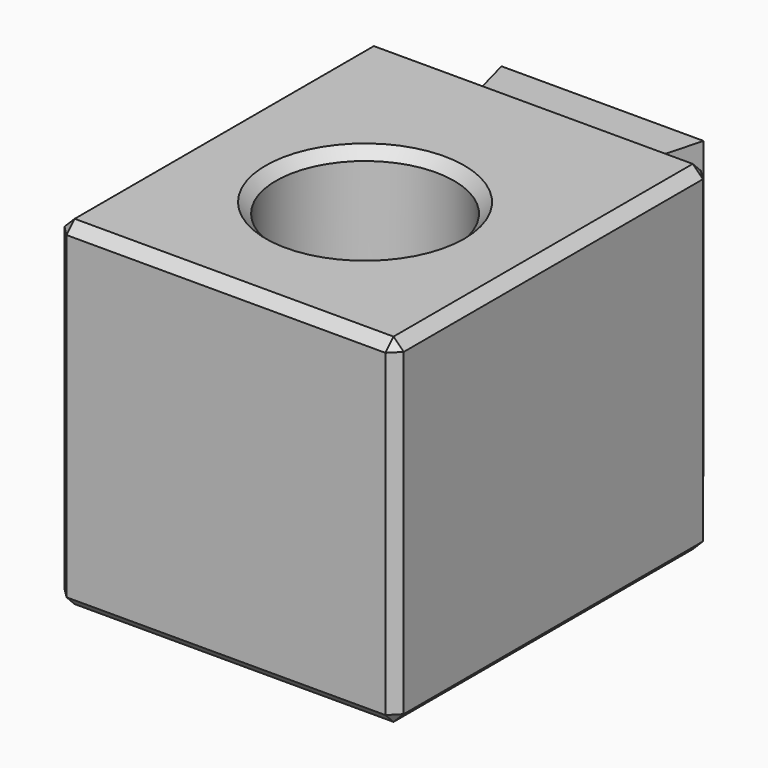
from build123d import *

# Parameters (mm, degrees)
F2_R     = 5.25
F3_DEPTH = 20
F4_DEPTH = 18
F5_SIZE  = 0.6


# Not quite as in the source:
# - a feature names something its author has since deleted; it is built from what else it names


with BuildPart() as f3:
    # F2 (on Top) → F3 (new body)
    with BuildSketch(Plane.XY):
        Polygon((5.25, 23.25), (0, 23.25), (0, 0), (20, 0), (20, 23.25), (14.75, 23.25), align=None)
        with Locations((10, 10.25)):
            Circle(F2_R, mode=Mode.SUBTRACT)
    extrude(amount=F3_DEPTH)

    # F2 (on Top) → F4 (join)
    with BuildSketch(Plane.XY):
        Polygon((4.0442286341, 27.75), (5.25, 23.25), (14.75, 23.25), (15.9557713659, 27.75), align=None)
    extrude(amount=F4_DEPTH)

    # F5
    f5_edges = [f3.edges().sort_by_distance(p)[0] for p in [
        (0, 11.625, 0),
        (10, 0, 0),
        (20, 11.625, 0),
        (17.375, 23.25, 0),
        (15.352886, 25.5, 0),
        (10, 27.75, 0),
        (4.647114, 25.5, 0),
        (2.625, 23.25, 0),
        (4.75, 10.25, 0),
        (10, 23.25, 20),
        (0, 11.625, 20),
        (10, 0, 20),
        (20, 11.625, 20),
        (4.75, 10.25, 20),
        (0, 0, 10),
        (20, 0, 10),
        (20, 23.25, 10),
    ]]
    chamfer(f5_edges, length=F5_SIZE)


solid = f3.part
